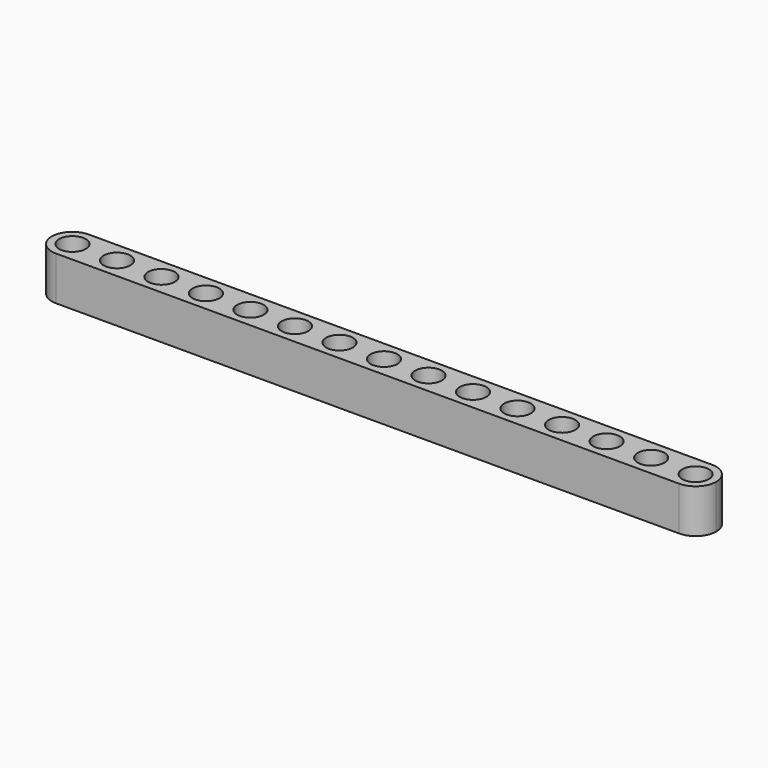
from build123d import *

# Parameters (mm, degrees)
F0_R        = 2.4
F1_DEPTH    = 7.88
F2_T1_DEPTH = 26.405


# Not quite as in the source:
# - a fillet or chamfer that OpenCascade refuses, or shapes differently, is made with other operations: its cross-section is extruded or revolved along the edge and cut away or added


with BuildPart() as f1:
    # F0 (on Top) → F1 (new body)
    with BuildSketch(Plane.XY):
        Polygon((30.9904916829, 1.6058013724), (-28.7195083171, 1.6058013724), (-88.4295083171, 1.6058013724), (-88.4295083171, -2.0891986276), (-88.4295083171, -5.7841986276), (-28.7195083171, -5.7841986276), (30.9904916829, -5.7841986276), (30.9904916829, -2.0891986276), align=None)
        with Locations((-84.7195083171, -2.0891986276)):
            Circle(F0_R, mode=Mode.SUBTRACT)
        with Locations((-76.7195083171, -2.0891986276)):
            Circle(F0_R, mode=Mode.SUBTRACT)
        with Locations((-68.7195083171, -2.0891986276)):
            Circle(F0_R, mode=Mode.SUBTRACT)
        with Locations((-60.7195083171, -2.0891986276)):
            Circle(F0_R, mode=Mode.SUBTRACT)
        with Locations((-52.7195083171, -2.0891986276)):
            Circle(F0_R, mode=Mode.SUBTRACT)
        with Locations((-44.7195083171, -2.0891986276)):
            Circle(F0_R, mode=Mode.SUBTRACT)
        with Locations((-36.7195083171, -2.0891986276)):
            Circle(F0_R, mode=Mode.SUBTRACT)
        with BuildLine():
            ThreePointArc((-28.7195083171, -4.4891986276), (-31.1195083171, -2.0891986276), (-28.7195083171, 0.3108013724))
            ThreePointArc((-28.7195083171, 0.3108013724), (-26.3195083171, -2.0891986276), (-28.7195083171, -4.4891986276))
        make_face(mode=Mode.SUBTRACT)
        with Locations((-20.7195083171, -2.0891986276)):
            Circle(F0_R, mode=Mode.SUBTRACT)
        with Locations((-12.7195083171, -2.0891986276)):
            Circle(F0_R, mode=Mode.SUBTRACT)
        with Locations((-4.7195083171, -2.0891986276)):
            Circle(F0_R, mode=Mode.SUBTRACT)
        with Locations((3.2804916829, -2.0891986276)):
            Circle(F0_R, mode=Mode.SUBTRACT)
        with Locations((11.2804916829, -2.0891986276)):
            Circle(F0_R, mode=Mode.SUBTRACT)
        with Locations((19.2804916829, -2.0891986276)):
            Circle(F0_R, mode=Mode.SUBTRACT)
        with Locations((27.2804916829, -2.0891986276)):
            Circle(F0_R, mode=Mode.SUBTRACT)
    extrude(amount=F1_DEPTH)

    # F2: fillet of radius 3.705 on 4 edges, made by hand

    # F2_s2 → F2_t1 (cut)
    with BuildSketch(Plane.XY.offset(-9.2625)):
        with BuildLine():
            ThreePointArc((27.2854916829, 1.6058013724), (29.9053223072, 0.5206319967), (30.9904916829, -2.0991986276))
            Line((30.9904916829, -2.0991986276), (30.9904916829, 1.6058013724))
            Line((30.9904916829, 1.6058013724), (27.2854916829, 1.6058013724))
        make_face()
        with BuildLine():
            ThreePointArc((27.2854916829, -5.7841986276), (29.9053223072, -4.6990292519), (30.9904916829, -2.0791986276))
            Line((30.9904916829, -2.0791986276), (30.9904916829, -5.7841986276))
            Line((30.9904916829, -5.7841986276), (27.2854916829, -5.7841986276))
        make_face()
        with BuildLine():
            ThreePointArc((-84.7245083171, 1.6058013724), (-87.3443389413, 0.5206319967), (-88.4295083171, -2.0991986276))
            Line((-88.4295083171, -2.0991986276), (-88.4295083171, 1.6058013724))
            Line((-88.4295083171, 1.6058013724), (-84.7245083171, 1.6058013724))
        make_face()
        with BuildLine():
            ThreePointArc((-84.7245083171, -5.7841986276), (-87.3443389413, -4.6990292519), (-88.4295083171, -2.0791986276))
            Line((-88.4295083171, -2.0791986276), (-88.4295083171, -5.7841986276))
            Line((-88.4295083171, -5.7841986276), (-84.7245083171, -5.7841986276))
        make_face()
    extrude(amount=F2_T1_DEPTH, mode=Mode.SUBTRACT)


solid = f1.part
